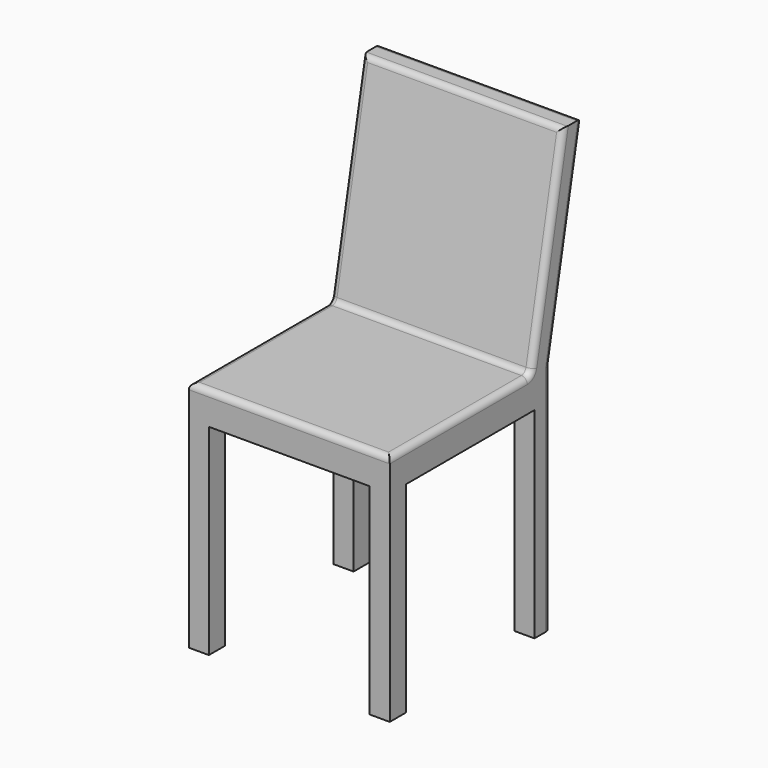
from build123d import *

# Parameters (mm, degrees)
F0_W            = 500
F0_H            = 500
F1_DEPTH        = 80
F2_W            = 50
F2_H            = 50
F3_DEPTH        = 500
F3_COPIES_COUNT = 4
F6_DEPTH        = 250
F7_R            = 15


# Not quite as in the source:
# - a pattern or mirror of a feature is missing from the dataset's text; its kind, count and spacing are read off the source's solid


with BuildPart() as f1:
    # F0 (on Top) → F1 (new body)
    with BuildSketch(Plane.XY):
        Rectangle(F0_W, F0_H)
    extrude(amount=F1_DEPTH)

    # F2 (on face) → F3 (join)
    with BuildSketch(Plane(origin=(0, 0, 0), x_dir=(1, 0, 0), z_dir=(0, 0, -1))):
        with Locations((-225, 225)):
            Rectangle(F2_W, F2_H)
    f3 = extrude(amount=F3_DEPTH)

    # F3_copies: F3 ×4 about axis
    f3_copies_axis = Axis((0, 0, 0), (0, 0, 1))
    for i in range(1, F3_COPIES_COUNT):
        add(f3.rotate(f3_copies_axis, i * 360 / F3_COPIES_COUNT))

    # F5 (on Right) → F6 (join, symmetric)
    with BuildSketch(Plane.YZ):
        Polygon((290, 580), (190, 80), (250, 80), (350, 580), align=None)
    extrude(amount=F6_DEPTH, both=True)

    # F7
    f7_edges = [f1.edges().sort_by_distance(p)[0] for p in [
        (0, -250, 80),
        (-250, -30, 80),
        (0, 190, 80),
        (250, -30, 80),
        (-250, 240, 330),
        (250, 240, 330),
        (0, 290, 580),
        (0, 250, 80),
        (-250, 300, 330),
        (0, 350, 580),
        (250, 300, 330),
        (250, 250, -210),
        (-250, 250, -210),
    ]]
    fillet(f7_edges, radius=F7_R)


solid = f1.part
